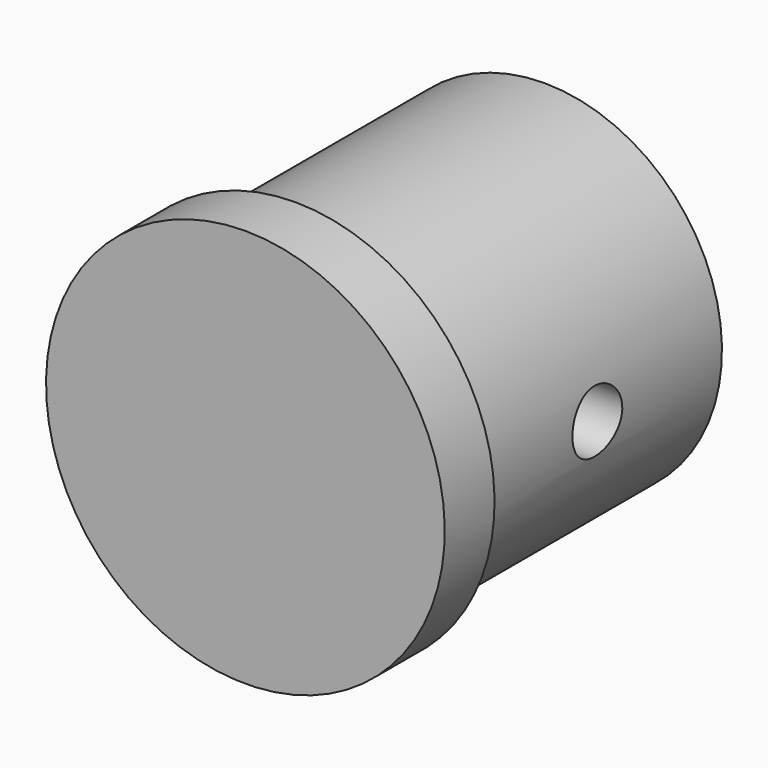
from build123d import *

# Parameters (mm, degrees)
F6_D     = 2
F6_DEPTH = 5.7
F6_TIP   = 0.600860619


# Not quite as in the source:
# - a feature names something its author has since deleted; it is built from what else it names


with BuildPart() as f3:
    # F2 (on Right) → F3 (revolve)
    with BuildSketch(Plane.YZ):
        Polygon((0, 0), (12, 0), (12, 5.7), (2, 5.7), (2, 6.4), (0, 6.4), align=None)
    revolve(axis=Axis((0, 5.7350749573, 0), (0, -1, 0)))

    # F6
    with Locations(Plane.YZ.offset(5.7)):
        with Locations((7, 0)):
            Hole(F6_D / 2, depth=F6_DEPTH)
            with Locations((0, 0, -(F6_DEPTH + F6_TIP / 2))):  # 118° drill point
                Cone(0, F6_D / 2, F6_TIP, mode=Mode.SUBTRACT)


solid = f3.part
